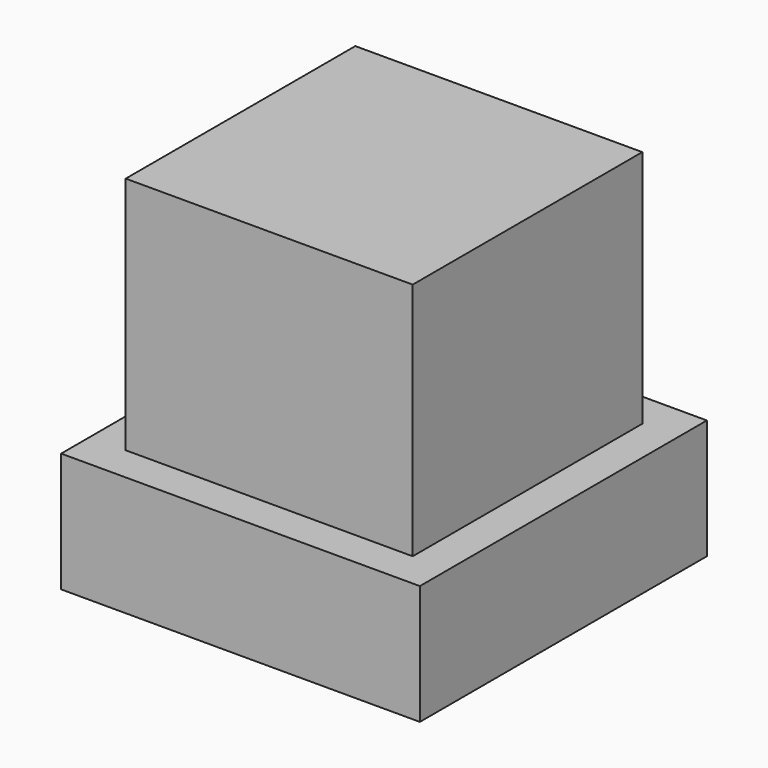
from build123d import *

# Parameters (mm, degrees)
F0_W     = 15
F0_H     = 15
F0_W_2   = 12
F0_H_2   = 12
F1_DEPTH = 5
F2_DEPTH = 10


with BuildPart() as f1:
    # F0 (on Top) → F1 (new body)
    with BuildSketch(Plane.XY):
        Rectangle(F0_W, F0_H)
        Rectangle(F0_W_2, F0_H_2, mode=Mode.SUBTRACT)
        Rectangle(F0_W_2, F0_H_2)
    extrude(amount=-F1_DEPTH)

    # F0 (on Top) → F2 (join)
    with BuildSketch(Plane.XY):
        Rectangle(F0_W_2, F0_H_2)
    extrude(amount=F2_DEPTH)


solid = f1.part
